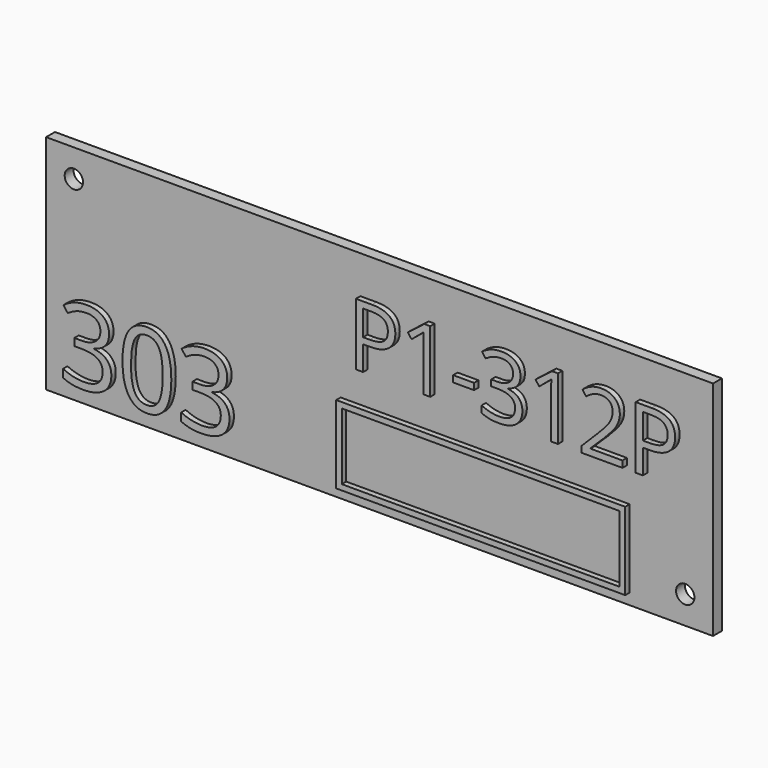
from build123d import *

# Parameters (mm, degrees)
F0_W         = 120
F0_H         = 40
F1_DEPTH     = 2
F3_D         = 3.3
F4_TEXT_SIZE = 15.681149951
F5_DEPTH     = 1
F6_TEXT_SIZE = 18.5894526641
F7_DEPTH     = 1
F8_W         = 52
F8_H         = 14
F8_W_2       = 49.99999962
F8_H_2       = 11.99999962
F9_DEPTH     = 1


# Not quite as in the source:
# - Text() gives the source's letters only with a copy of the font that has no kerning and outlines rounded to 1/6400 em; it was checked with that copy


with BuildPart() as f1:
    # F0 (on Front) → F1 (new body)
    with BuildSketch(Plane.XZ):
        Rectangle(F0_W, F0_H)
    extrude(amount=F1_DEPTH)

    # F3 (through all)
    with Locations(Plane.XZ.offset(2)):
        with Locations((-55, 15), (55, -15)):
            Hole(F3_D / 2)

    # F4 (on face) → F5 (join)
    with BuildSketch(Plane.XZ.offset(2)):
        with Locations((-5, 2)):
            Text('P1-312P', F4_TEXT_SIZE, font='Open Sans', text_align=(TextAlign.LEFT, TextAlign.BOTTOM))
    extrude(amount=F5_DEPTH)

    # F6 (on face) → F7 (join)
    with BuildSketch(Plane.XZ.offset(2)):
        with Locations((-57, -17)):
            Text('303', F6_TEXT_SIZE, font='Open Sans', text_align=(TextAlign.LEFT, TextAlign.BOTTOM))
    extrude(amount=F7_DEPTH)

    # F8 (on face) → F9 (join)
    with BuildSketch(Plane.XZ.offset(2)):
        with Locations((19, -11)):
            Rectangle(F8_W, F8_H)
        with Locations((19, -11)):
            Rectangle(F8_W_2, F8_H_2, mode=Mode.SUBTRACT)
    extrude(amount=F9_DEPTH)


solid = f1.part
